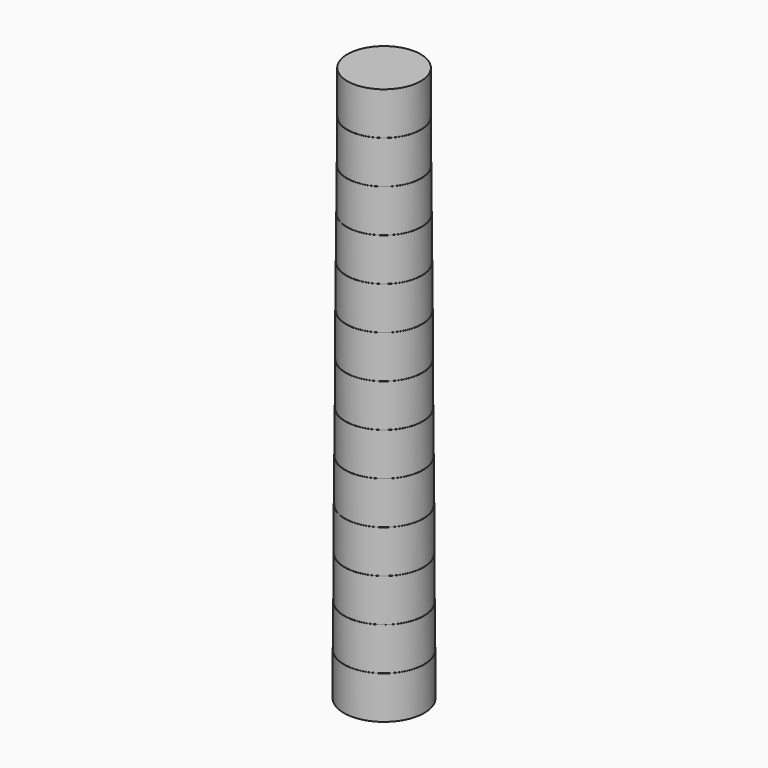
from build123d import *

# Parameters (mm, degrees)
F0_R      = 6.6
F1_DEPTH  = 7
F2_R      = 6.55
F3_DEPTH  = 7
F4_R      = 6.5
F5_DEPTH  = 7
F6_R      = 6.45
F7_DEPTH  = 7
F8_R      = 6.4
F9_DEPTH  = 7
F10_R     = 6.35
F11_DEPTH = 7
F12_R     = 6.3
F13_DEPTH = 7
F14_R     = 6.25
F15_DEPTH = 7
F16_R     = 6.2
F17_DEPTH = 7
F18_R     = 6.15
F19_DEPTH = 7
F20_R     = 6.1
F21_DEPTH = 7
F22_R     = 6.05
F23_DEPTH = 7
F24_R     = 6
F25_DEPTH = 7


# Not quite as in the source:
# - a feature of the source that left no trace in its solid (it failed there, or was rolled back) is left out


with BuildPart() as f1:
    # F0 (on Top) → F1 (new body)
    with BuildSketch(Plane.XY):
        Circle(F0_R)
    extrude(amount=F1_DEPTH)

    # F2 (on face) → F3 (join)
    with BuildSketch(Plane.XY.offset(7)):
        Circle(F2_R)
    extrude(amount=F3_DEPTH)

    # F4 (on face) → F5 (join)
    with BuildSketch(Plane.XY.offset(14)):
        Circle(F4_R)
    extrude(amount=F5_DEPTH)

    # F6 (on face) → F7 (join)
    with BuildSketch(Plane.XY.offset(21)):
        Circle(F6_R)
    extrude(amount=F7_DEPTH)

    # F8 (on face) → F9 (join)
    with BuildSketch(Plane.XY.offset(28)):
        Circle(F8_R)
    extrude(amount=F9_DEPTH)

    # F10 (on face) → F11 (join)
    with BuildSketch(Plane.XY.offset(35)):
        Circle(F10_R)
    extrude(amount=F11_DEPTH)

    # F12 (on face) → F13 (join)
    with BuildSketch(Plane.XY.offset(42)):
        Circle(F12_R)
    extrude(amount=F13_DEPTH)

    # F14 (on face) → F15 (join)
    with BuildSketch(Plane.XY.offset(49)):
        Circle(F14_R)
    extrude(amount=F15_DEPTH)

    # F16 (on face) → F17 (join)
    with BuildSketch(Plane.XY.offset(56)):
        Circle(F16_R)
    extrude(amount=F17_DEPTH)

    # F18 (on face) → F19 (join)
    with BuildSketch(Plane.XY.offset(63)):
        Circle(F18_R)
    extrude(amount=F19_DEPTH)

    # F20 (on face) → F21 (join)
    with BuildSketch(Plane.XY.offset(70)):
        Circle(F20_R)
    extrude(amount=F21_DEPTH)

    # F22 (on face) → F23 (join)
    with BuildSketch(Plane.XY.offset(77)):
        Circle(F22_R)
    extrude(amount=F23_DEPTH)

    # F24 (on face) → F25 (join)
    with BuildSketch(Plane.XY.offset(84)):
        Circle(F24_R)
    extrude(amount=F25_DEPTH)


solid = f1.part
